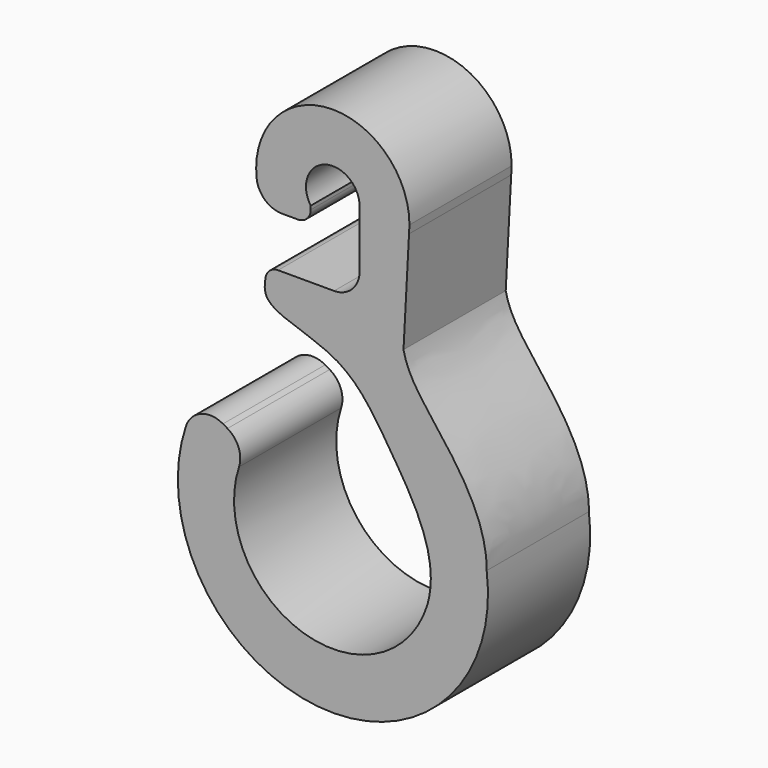
from build123d import *

# Parameters (mm, degrees)
F1_DEPTH = 10
F2_R     = 1
F3_R     = 2


# Not quite as in the source:
# - two fillets or chamfers of one size are made in one step
# - a feature names something its author has since deleted; it is built from what else it names


with BuildPart() as f1:
    # F0 (on Front) → F1 (new body)
    with BuildSketch(Plane.XZ):
        with BuildLine():
            ThreePointArc((-1.7285399627, -1.1925391387), (-0.6245262518, 2.0049855263), (2.1, 0))
            Line((2.1, 0), (2.1, -6.4722087772))
            Line((2.1, -6.4722087772), (-1.7285399627, -6.4722087772))
            Line((-1.7285399627, -6.4722087772), (-5.1270676777, -6.4722087772))
            add(Edge.make_bspline(
                [(-5.1270676777, -6.4722087772), (-5.2022797508, -7.1671189286), (-6.0866195882, -9.4345123751), (1.027351741, -10.4770430063), (4.526556097, -16.11453384), (8.4301587847, -22.1647756383), (7.4084669429, -25.7151645559)],
                knots=[0, 0, 0, 0, 0.1536701078, 0.4002962667, 0.6726958228, 1, 1, 1, 1], degree=3))
            ThreePointArc((7.4084669429, -25.7151645559), (-3.085024735, -30.5342112997), (-6.6922515438, -19.5649590981))
            Line((-6.6922515438, -19.5649590981), (-10.5016801666, -17.3630853307))
            ThreePointArc((-10.5016801666, -17.3630853307), (-2.3664943525, -35.3449464187), (12.0481319901, -21.8635843278))
            add(Edge.make_bspline(
                [(5.535574435, -8.7558477202), (5.8434484166, -10.2656725536), (7.9936891439, -13.1024488577), (12.074048333, -18.3231807373), (12.0481319901, -21.8635843278)],
                knots=[0, 0, 0, 0, 0.4156437378, 1, 1, 1, 1], degree=3))
            Line((5.535574435, -8.7558477202), (5.9663335796, -0.6347153824))
            Line((5.9663335796, -0.6347153824), (6, 0))
            ThreePointArc((6, 0), (-1.2645054368, 5.8652387846), (-5.4670086667, -2.4722087772))
            Line((-5.4670086667, -2.4722087772), (-1.7285399627, -2.4722087772))
            Line((-1.7285399627, -2.4722087772), (-1.7285399627, -1.1925391387))
        make_face()
    extrude(amount=F1_DEPTH)

    # F2
    f2_edges = [f1.edges().sort_by_distance(p)[0] for p in [
        (-1.72854, -5, -2.472209),
        (-5.127068, -5, -6.472209),
    ]]
    fillet(f2_edges, radius=F2_R)

    # F3
    f3_edges = [f1.edges().sort_by_distance(p)[0] for p in [
        (-10.50168, -5, -17.363085),
        (-6.692252, -5, -19.564959),
        (-5.467009, -5, -2.472209),
        (2.1, -5, -6.472209),
    ]]
    fillet(f3_edges, radius=F3_R)


solid = f1.part
